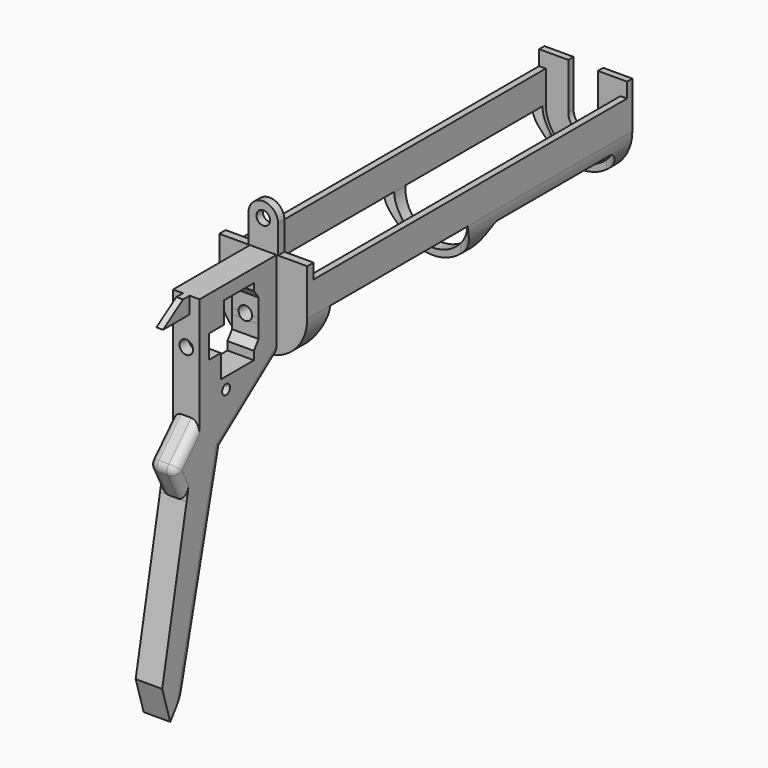
from build123d import *

# Parameters (mm, degrees)
F1_DEPTH      = 245
F3_DEPTH      = 26.501
F5_DEPTH      = 4
F7_DEPTH      = 4.8
F8_R          = 4.1
F9_DEPTH      = 245.0010001
F10_W         = 17.5768885165
F10_H         = 9
F11_DEPTH     = 4
F14_DEPTH     = 8
F16_DEPTH     = 34.5010001
F17_DEPTH     = 86.1370478401
F18_R         = 3
F19_DEPTH     = 25
F20_R         = 5
F21_T4_DEPTH  = 36.9491511405
F21_T9_DEPTH  = 36.9491511405
F21_T14_DEPTH = 141.5
F21_T19_DEPTH = 76
F21_T25_DEPTH = 141.5
F21_T30_DEPTH = 76
F21_T34_ANGLE = 70.7624369156
F21_T38_DEPTH = 29.9491511405
F21_T41_ANGLE = 70.7624369156
F21_T45_DEPTH = 29.9491511405
F21_T51_DEPTH = 76
F21_T55_DEPTH = 141.5
F21_T62_DEPTH = 76
F21_T66_DEPTH = 141.5
F22_DEPTH     = 2


# Not quite as in the source:
# - a fillet or chamfer that OpenCascade refuses, or shapes differently, is made with other operations: its cross-section is extruded or revolved along the edge and cut away or added
# - a feature names something its author has since deleted; it is built from what else it names


with BuildPart() as f1:
    # F0 (on Front) → F1 (new body)
    with BuildSketch(Plane.XZ):
        with BuildLine():
            Line((-22.5, 0), (-22.5, 19))
            Line((-22.5, 19), (-26.5, 19))
            Line((-26.5, 19), (-26.5, 0))
            ThreePointArc((-26.5, 0), (0, -26.5), (26.5, 0))
            Line((26.5, 0), (26.5, 19))
            Line((26.5, 19), (22.5, 19))
            Line((22.5, 19), (22.5, 0))
            ThreePointArc((22.5, 0), (0, -22.5), (-22.5, 0))
        make_face()
    extrude(amount=F1_DEPTH)

    # F2 (on Top) → F3 (cut, through all)
    with BuildSketch(Plane.XY):
        with BuildLine():
            Line((17.2196690738, -117.5267648697), (-18.8738906384, -117.5267648697))
            ThreePointArc((-18.8738906384, -117.5267648697), (-25.9449584502, -120.4556970578), (-28.8738906384, -127.5267648697))
            Line((-28.8738906384, -127.5267648697), (-28.8738906384, -224.1310429573))
            ThreePointArc((-28.8738906384, -224.1310429573), (-25.9449584502, -231.2021107692), (-18.8738906384, -234.1310429573))
            Line((-18.8738906384, -234.1310429573), (17.2196690738, -234.1310429573))
            ThreePointArc((17.2196690738, -234.1310429573), (24.2907368857, -231.2021107692), (27.2196690738, -224.1310429573))
            Line((27.2196690738, -224.1310429573), (27.2196690738, -127.5267648697))
            ThreePointArc((27.2196690738, -127.5267648697), (24.2907368857, -120.4556970578), (17.2196690738, -117.5267648697))
        make_face()
        with BuildLine():
            Line((15.6445064396, -5.7718827203), (-18.8738906384, -5.7718827203))
            ThreePointArc((-18.8738906384, -5.7718827203), (-25.9449584502, -8.7008149084), (-28.8738906384, -15.7718827203))
            Line((-28.8738906384, -15.7718827203), (-28.8738906384, -100.5394262075))
            ThreePointArc((-28.8738906384, -100.5394262075), (-25.9449584502, -107.6104940194), (-18.8738906384, -110.5394262075))
            Line((-18.8738906384, -110.5394262075), (15.6445064396, -110.5394262075))
            ThreePointArc((15.6445064396, -110.5394262075), (22.7155742514, -107.6104940194), (25.6445064396, -100.5394262075))
            Line((25.6445064396, -100.5394262075), (25.6445064396, -15.7718827203))
            ThreePointArc((25.6445064396, -15.7718827203), (22.7155742514, -8.7008149084), (15.6445064396, -5.7718827203))
        make_face()
    extrude(amount=-F3_DEPTH, mode=Mode.SUBTRACT)

    # F4 (on face) → F5 (join)
    with BuildSketch(Plane(origin=(0, 0, 0), x_dir=(-1, 0, 0), z_dir=(0, 1, 0))):
        with BuildLine():
            Line((-8.9231114835, 19), (-22.5, 19))
            Line((-22.5, 19), (-22.5, 0))
            ThreePointArc((-22.5, 0), (0, -22.5), (22.5, 0))
            Line((22.5, 0), (22.5, 19))
            Line((22.5, 19), (8.9231114835, 19))
            Line((8.9231114835, 19), (8.9231114835, 0))
            ThreePointArc((8.9231114835, 0), (0, -8.9231114835), (-8.9231114835, 0))
            Line((-8.9231114835, 0), (-8.9231114835, 19))
        make_face()
    extrude(amount=-F5_DEPTH)

    # F6 (on face) → F7 (join)
    with BuildSketch(Plane.XZ.offset(245)):
        with BuildLine():
            Line((-26.5, 28), (-26.5, 19))
            Line((-26.5, 19), (-22.5, 19))
            Line((-22.5, 19), (-22.5, 0))
            ThreePointArc((-22.5, 0), (0, -22.5), (22.5, 0))
            Line((22.5, 0), (22.5, 19))
            Line((22.5, 19), (26.5, 19))
            Line((26.5, 19), (26.5, 28))
            Line((26.5, 28), (8.9231114835, 28))
            Line((8.9231114835, 28), (8.9231114835, 44.9963948429))
            ThreePointArc((8.9231114835, 44.9963948429), (0, 53.9195063263), (-8.9231114835, 44.9963948429))
            Line((-8.9231114835, 44.9963948429), (-8.9231114835, 28))
            Line((-8.9231114835, 28), (-26.5, 28))
        make_face()
    extrude(amount=-F7_DEPTH)

    # F8 (on face) → F9 (cut, through all)
    with BuildSketch(Plane.XZ.offset(245)):
        with Locations((0, 44.9963948429)):
            Circle(F8_R)
        Circle(F8_R)
    extrude(amount=-F9_DEPTH, mode=Mode.SUBTRACT)

    # F10 (on face) → F11 (join)
    with BuildSketch(Plane(origin=(0, 0, 0), x_dir=(-1, 0, 0), z_dir=(0, 1, 0))):
        with Locations((-17.7115557417, 23.5)):
            Rectangle(F10_W, F10_H)
        with Locations((17.7115557417, 23.5)):
            Rectangle(F10_W, F10_H)
    extrude(amount=-F11_DEPTH)

    # F13 (on offset) → F14 (join, symmetric)
    with BuildSketch(Plane(origin=(0, 0, 0), x_dir=(0, -1, 0), z_dir=(-1, 0, 0))):
        Polygon((245, 28.0010560152), (245, -26.5), (285.7996278066, -57.1004962516), (312.754499772, -170.4393019508), (325.0868223385, -187.2815242885), (331.1360478401, -167.302697897), (312.754499772, -75.4479333324), (322.3185739144, -56.7522523927), (302.9845754006, -36.4989439848), (302.9845754006, 18.0010560152), (302.9845754006, 28.0010560152), align=None)
    extrude(amount=F14_DEPTH, both=True)

    # F15 (on face) → F16 (cut, through all)
    with BuildSketch(Plane(origin=(-8, 0, 0), x_dir=(0, -1, 0), z_dir=(-1, 0, 0))):
        Polygon((284.4845754006, 20.0010560152), (262, 20.0010560152), (262, 15.7399242051), (258.5, 10.8665270327), (258.5, 0.1439954649), (258.501, 0.1439954649), (258.501, -3.3005413134), (258.5, -3.3005413134), (258.5, -11.1334729673), (262, -16.0068701397), (262, -20.9989439848), (287, -20.9989439848), (287, -6.9989439848), (295.9845754006, -6.9989439848), (295.9845754006, 7.0010560152), (284.4845754006, 7.0010560152), align=None)
    extrude(amount=-F16_DEPTH, mode=Mode.SUBTRACT)

    # F17 (cut, through all): a face of the model
    f17_faces = [f1.faces().sort_by_distance(p)[0] for p in [
        (0, -245, 0),
    ]]
    extrude(f17_faces, amount=-F17_DEPTH, mode=Mode.SUBTRACT)

    # F18 (on face) → F19 (cut)
    with BuildSketch(Plane(origin=(-8, 0, 0), x_dir=(0, -1, 0), z_dir=(-1, 0, 0))):
        with Locations((282.9845754006, -27.9989439848)):
            Circle(F18_R)
    extrude(amount=-F19_DEPTH, mode=Mode.SUBTRACT)

    # F20
    f20_edges = [f1.edges().sort_by_distance(p)[0] for p in [
        (0, -322.318574, -56.752252),
    ]]
    fillet(f20_edges, radius=F20_R)

    # F21: fillet of radius 5 on 6 edges, made by hand


with BuildPart() as f21_tool2:
    # F21_s3 → F21_t4 (new body)
    with BuildSketch(Plane(origin=(0, -179.5720063651, -188.1104533936), x_dir=(1, 0, 0), z_dir=(0, 0.6904999469, 0.7233324431))):
        with BuildLine():
            ThreePointArc((-3, -193.9560542744), (-6.5355339059, -192.4915881803), (-8, -188.9560542744))
            Line((-8, -188.9560542744), (-8, -193.9560542744))
            Line((-8, -193.9560542744), (-3, -193.9560542744))
        make_face()
    extrude(amount=F21_T4_DEPTH)

    split(bisect_by=Plane.XZ.offset(302.9845754006), keep=Keep.TOP)


with BuildPart() as f1_1:
    add(f1.part)

    # F21_t1: cut F21_tool2
    add(f21_tool2.part, mode=Mode.SUBTRACT)


with BuildPart() as f21_tool7:
    # F21_s8 → F21_t9 (new body)
    with BuildSketch(Plane(origin=(0, -179.5720063651, -188.1104533936), x_dir=(1, 0, 0), z_dir=(0, 0.6904999469, 0.7233324431))):
        with BuildLine():
            ThreePointArc((8, -188.9560542744), (6.5355339059, -192.4915881803), (3, -193.9560542744))
            Line((3, -193.9560542744), (8, -193.9560542744))
            Line((8, -193.9560542744), (8, -188.9560542744))
        make_face()
    extrude(amount=F21_T9_DEPTH)

    split(bisect_by=Plane.XZ.offset(302.9845754006), keep=Keep.TOP)


with BuildPart() as f1_2:
    add(f1_1.part)

    # F21_t6: cut F21_tool7
    add(f21_tool7.part, mode=Mode.SUBTRACT)


with BuildPart() as f21_tool12:
    # F21_s13 → F21_t14 (new body)
    with BuildSketch(Plane(origin=(0, -25.2605801908, -106.2147130121), x_dir=(1, 0, 0), z_dir=(0, -0.2313722915, -0.972865285))):
        with BuildLine():
            ThreePointArc((-3, 264.8330636846), (-6.5355339059, 266.2975297786), (-8, 269.8330636846))
            Line((-8, 269.8330636846), (-8, 264.8330636846))
            Line((-8, 264.8330636846), (-3, 264.8330636846))
        make_face()
    extrude(amount=F21_T14_DEPTH)

    split(bisect_by=Plane(origin=(0, -75.4827705215, 100.6411437829), x_dir=(1, 0, 0), z_dir=(0, 0.6000097304, -0.7999927021)), keep=Keep.TOP)


with BuildPart() as f1_3:
    add(f1_2.part)

    # F21_t11: cut F21_tool12
    add(f21_tool12.part, mode=Mode.SUBTRACT)


with BuildPart() as f21_tool17:
    # F21_s18 → F21_t19 (new body)
    with BuildSketch(Plane(origin=(0, -159.5173207024, -119.6410221526), x_dir=(1, 0, 0), z_dir=(0, -0.7999927021, -0.6000097304))):
        with BuildLine():
            ThreePointArc((-3, 125.8025773485), (-6.5355339059, 127.2670434426), (-8, 130.8025773485))
            Line((-8, 130.8025773485), (-8, 125.8025773485))
            Line((-8, 125.8025773485), (-3, 125.8025773485))
        make_face()
    extrude(amount=F21_T19_DEPTH)

    split(bisect_by=Plane.XZ.offset(245), keep=Keep.TOP)

    split(bisect_by=Plane(origin=(0, -257.6468939714, 61.2750328226), x_dir=(1, 0, 0), z_dir=(0, 0.972865285, -0.2313722915)), keep=Keep.TOP)


with BuildPart() as f1_4:
    add(f1_3.part)

    # F21_t16: cut F21_tool17
    add(f21_tool17.part, mode=Mode.SUBTRACT)


with BuildPart() as f21_tool23:
    # F21_s24 → F21_t25 (new body)
    with BuildSketch(Plane(origin=(0, -25.2605801908, -106.2147130121), x_dir=(1, 0, 0), z_dir=(0, -0.2313722915, -0.972865285))):
        with BuildLine():
            ThreePointArc((8, 269.8330636846), (6.5355339059, 266.2975297786), (3, 264.8330636846))
            Line((3, 264.8330636846), (8, 264.8330636846))
            Line((8, 264.8330636846), (8, 269.8330636846))
        make_face()
    extrude(amount=F21_T25_DEPTH)

    split(bisect_by=Plane(origin=(0, -75.4827705215, 100.6411437829), x_dir=(1, 0, 0), z_dir=(0, 0.6000097304, -0.7999927021)), keep=Keep.TOP)


with BuildPart() as f1_5:
    add(f1_4.part)

    # F21_t22: cut F21_tool23
    add(f21_tool23.part, mode=Mode.SUBTRACT)


with BuildPart() as f21_tool28:
    # F21_s29 → F21_t30 (new body)
    with BuildSketch(Plane(origin=(0, -159.5173207024, -119.6410221526), x_dir=(1, 0, 0), z_dir=(0, -0.7999927021, -0.6000097304))):
        with BuildLine():
            ThreePointArc((8, 130.8025773485), (6.5355339059, 127.2670434426), (3, 125.8025773485))
            Line((3, 125.8025773485), (8, 125.8025773485))
            Line((8, 125.8025773485), (8, 130.8025773485))
        make_face()
    extrude(amount=F21_T30_DEPTH)

    split(bisect_by=Plane.XZ.offset(245), keep=Keep.TOP)

    split(bisect_by=Plane(origin=(0, -257.6468939714, 61.2750328226), x_dir=(1, 0, 0), z_dir=(0, 0.972865285, -0.2313722915)), keep=Keep.TOP)


with BuildPart() as f1_6:
    add(f1_5.part)

    # F21_t27: cut F21_tool28
    add(f21_tool28.part, mode=Mode.SUBTRACT)

    # F21_s33 → F21_t34 (revolve, cut)
    with BuildSketch(Plane(origin=(0, -179.5720063651, -188.1104533936), x_dir=(1, 0, 0), z_dir=(0, 0.6904999469, 0.7233324431))):
        with BuildLine():
            ThreePointArc((8, -188.9560542744), (6.5355339059, -192.4915881803), (3, -193.9560542744))
            Line((3, -193.9560542744), (8, -193.9560542744))
            Line((8, -193.9560542744), (8, -188.9560542744))
        make_face()
    revolve(axis=Axis((8, -316.2500507497, -57.6363079466), (1, 0, 0)), revolution_arc=F21_T34_ANGLE, mode=Mode.SUBTRACT)


with BuildPart() as f21_tool36:
    # F21_s37 → F21_t38 (new body)
    with BuildSketch(Plane(origin=(0, -28.5871853634, 55.8817182469), x_dir=(1, 0, 0), z_dir=(0, -0.455432102, 0.8902705209))):
        with BuildLine():
            ThreePointArc((8, -307.7975223082), (6.5355339059, -311.3330562142), (3, -312.7975223082))
            Line((3, -312.7975223082), (8, -312.7975223082))
            Line((8, -312.7975223082), (8, -307.7975223082))
        make_face()
    extrude(amount=F21_T38_DEPTH)

    split(bisect_by=Plane(origin=(0, -286.1951941692, 57.27205054), x_dir=(1, 0, 0), z_dir=(0, -0.9805589188, 0.1962248881)), keep=Keep.TOP)


with BuildPart() as f1_7:
    add(f1_6.part)

    # F21_t35: cut F21_tool36
    add(f21_tool36.part, mode=Mode.SUBTRACT)

    # F21_s40 → F21_t41 (revolve, cut)
    with BuildSketch(Plane(origin=(0, -179.5720063651, -188.1104533936), x_dir=(1, 0, 0), z_dir=(0, 0.6904999469, 0.7233324431))):
        with BuildLine():
            ThreePointArc((-3, -193.9560542744), (-6.5355339059, -192.4915881803), (-8, -188.9560542744))
            Line((-8, -188.9560542744), (-8, -193.9560542744))
            Line((-8, -193.9560542744), (-3, -193.9560542744))
        make_face()
    revolve(axis=Axis((-8, -316.2500507497, -57.6363079466), (1, 0, 0)), revolution_arc=F21_T41_ANGLE, mode=Mode.SUBTRACT)


with BuildPart() as f21_tool43:
    # F21_s44 → F21_t45 (new body)
    with BuildSketch(Plane(origin=(0, -28.5871853634, 55.8817182469), x_dir=(1, 0, 0), z_dir=(0, -0.455432102, 0.8902705209))):
        with BuildLine():
            ThreePointArc((-3, -312.7975223082), (-6.5355339059, -311.3330562142), (-8, -307.7975223082))
            Line((-8, -307.7975223082), (-8, -312.7975223082))
            Line((-8, -312.7975223082), (-3, -312.7975223082))
        make_face()
    extrude(amount=F21_T45_DEPTH)

    split(bisect_by=Plane(origin=(0, -286.1951941692, 57.27205054), x_dir=(1, 0, 0), z_dir=(0, -0.9805589188, 0.1962248881)), keep=Keep.TOP)


with BuildPart() as f1_8:
    add(f1_7.part)

    # F21_t42: cut F21_tool43
    add(f21_tool43.part, mode=Mode.SUBTRACT)


with BuildPart() as f21_tool49:
    # F21_s50 → F21_t51 (new body)
    with BuildSketch(Plane(origin=(0, -159.5173207024, -119.6410221526), x_dir=(1, 0, 0), z_dir=(0, -0.7999927021, -0.6000097304))):
        with BuildLine():
            ThreePointArc((-3, 125.8025773485), (-6.5355339059, 127.2670434426), (-8, 130.8025773485))
            Line((-8, 130.8025773485), (-8, 125.8025773485))
            Line((-8, 125.8025773485), (-3, 125.8025773485))
        make_face()
    extrude(amount=F21_T51_DEPTH)

    split(bisect_by=Plane(origin=(0, -257.6468939714, 61.2750328226), x_dir=(1, 0, 0), z_dir=(0, -0.972865285, 0.2313722915)), keep=Keep.TOP)


with BuildPart() as f21_tool53:
    # F21_s54 → F21_t55 (new body)
    with BuildSketch(Plane(origin=(0, -25.2605801908, -106.2147130121), x_dir=(1, 0, 0), z_dir=(0, -0.2313722915, -0.972865285))):
        with BuildLine():
            ThreePointArc((-3, 264.8330636846), (-6.5355339059, 266.2975297786), (-8, 269.8330636846))
            Line((-8, 269.8330636846), (-8, 264.8330636846))
            Line((-8, 264.8330636846), (-3, 264.8330636846))
        make_face()
    extrude(amount=F21_T55_DEPTH)

    split(bisect_by=Plane(origin=(0, -75.4827705215, 100.6411437829), x_dir=(1, 0, 0), z_dir=(0, -0.6000097304, 0.7999927021)), keep=Keep.TOP)


with BuildPart() as f21_tool49_1:
    add(f21_tool49.part)

    # F21_t57: intersect F21_tool53
    add(f21_tool53.part, mode=Mode.INTERSECT)


with BuildPart() as f1_9:
    add(f1_8.part)

    # F21_t47: cut F21_tool49
    add(f21_tool49_1.part, mode=Mode.SUBTRACT)


with BuildPart() as f21_tool60:
    # F21_s61 → F21_t62 (new body)
    with BuildSketch(Plane(origin=(0, -159.5173207024, -119.6410221526), x_dir=(1, 0, 0), z_dir=(0, -0.7999927021, -0.6000097304))):
        with BuildLine():
            ThreePointArc((8, 130.8025773485), (6.5355339059, 127.2670434426), (3, 125.8025773485))
            Line((3, 125.8025773485), (8, 125.8025773485))
            Line((8, 125.8025773485), (8, 130.8025773485))
        make_face()
    extrude(amount=F21_T62_DEPTH)

    split(bisect_by=Plane(origin=(0, -257.6468939714, 61.2750328226), x_dir=(1, 0, 0), z_dir=(0, -0.972865285, 0.2313722915)), keep=Keep.TOP)


with BuildPart() as f21_tool64:
    # F21_s65 → F21_t66 (new body)
    with BuildSketch(Plane(origin=(0, -25.2605801908, -106.2147130121), x_dir=(1, 0, 0), z_dir=(0, -0.2313722915, -0.972865285))):
        with BuildLine():
            ThreePointArc((8, 269.8330636846), (6.5355339059, 266.2975297786), (3, 264.8330636846))
            Line((3, 264.8330636846), (8, 264.8330636846))
            Line((8, 264.8330636846), (8, 269.8330636846))
        make_face()
    extrude(amount=F21_T66_DEPTH)

    split(bisect_by=Plane(origin=(0, -75.4827705215, 100.6411437829), x_dir=(1, 0, 0), z_dir=(0, -0.6000097304, 0.7999927021)), keep=Keep.TOP)


with BuildPart() as f21_tool60_1:
    add(f21_tool60.part)

    # F21_t68: intersect F21_tool64
    add(f21_tool64.part, mode=Mode.INTERSECT)


with BuildPart() as f1_10:
    add(f1_9.part)

    # F21_t58: cut F21_tool60
    add(f21_tool60_1.part, mode=Mode.SUBTRACT)

    # F13 (on offset) → F22 (join, symmetric)
    with BuildSketch(Plane(origin=(0, 0, 0), x_dir=(0, -1, 0), z_dir=(-1, 0, 0))):
        Polygon((307.9845754006, 28.0010560152), (302.9845754006, 28.0010560152), (302.9845754006, 18.0010560152), (322.9845754006, 18.0010560152), align=None)
    extrude(amount=F22_DEPTH, both=True)


solid = f1_10.part
